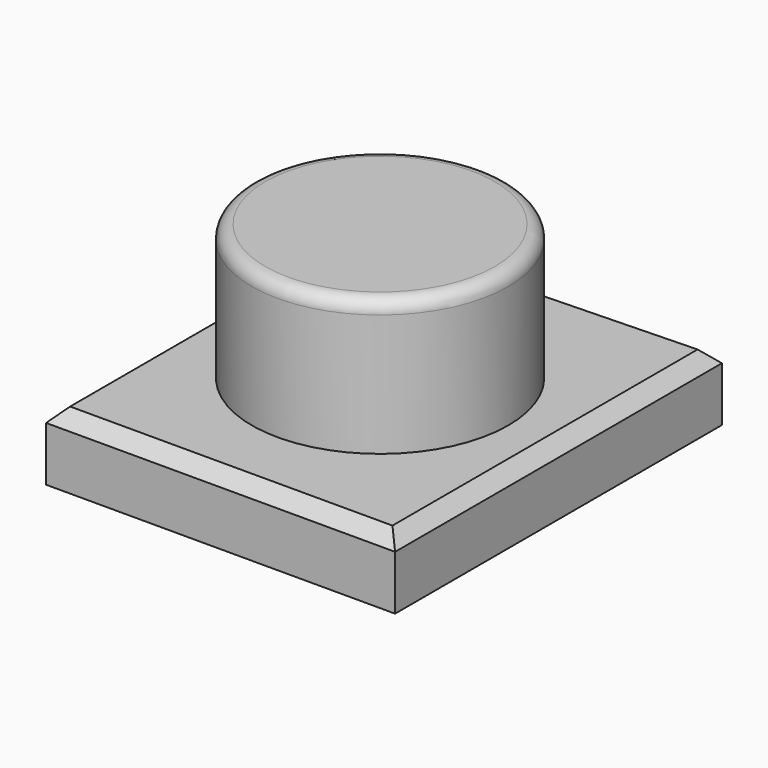
from build123d import *

# Parameters (mm, degrees)
F1_DEPTH = 25.4
F2_R     = 48.0357441032
F3_DEPTH = 50.8
F4_R     = 5
F5_SIZE  = 5


# Not quite as in the source:
# - the program builds the solid bodies; features that only make, move or delete a surface that nothing else refers to are left out


with BuildPart() as f1:
    # F0 (on Top) → F1 (new body)
    with BuildSketch(Plane.XY):
        Polygon((118.1704625487, 0), (-12.6199126244, -4.1209459305), (-12.6199126244, -153.0908346176), (118.1704625487, -153.0908346176), align=None)
    extrude(amount=F1_DEPTH)

    # F2 (on face) → F3 (join)
    with BuildSketch(Plane.XY.offset(25.4)):
        with Locations((51.9535280764, -77.3641169071)):
            Circle(F2_R)
    extrude(amount=F3_DEPTH)

    # F4
    f4_edges = [f1.edges().sort_by_distance(p)[0] for p in [
        (3.917784, -77.364117, 76.2),
    ]]
    fillet(f4_edges, radius=F4_R)

    # F5
    f5_edges = [f1.edges().sort_by_distance(p)[0] for p in [
        (118.170463, -76.545417, 25.4),
        (52.775275, -2.060473, 25.4),
        (-12.619913, -78.60589, 25.4),
        (52.775275, -153.090835, 25.4),
    ]]
    chamfer(f5_edges, length=F5_SIZE)


solid = f1.part
